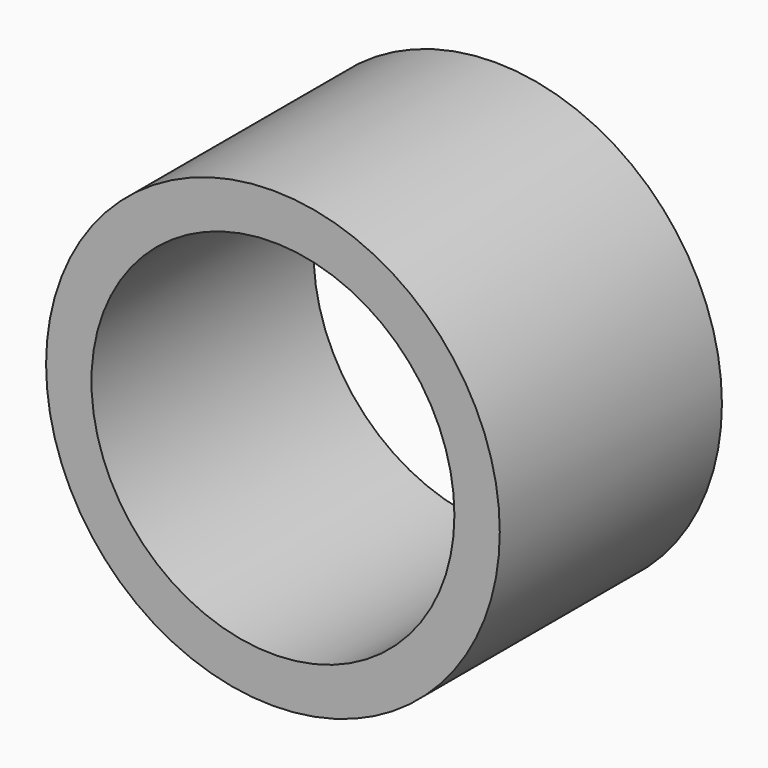
from build123d import *

# Parameters (mm, degrees)
F0_R     = 63.5
F0_R_2   = 50.8
F1_DEPTH = 77.724


# Not quite as in the source:
# - a feature names something its author has since deleted; it is built from what else it names


with BuildPart() as f1:
    # F0 (on Front) → F1 (new body)
    with BuildSketch(Plane.XZ):
        Circle(F0_R)
        Circle(F0_R_2, mode=Mode.SUBTRACT)
    extrude(amount=F1_DEPTH)


solid = f1.part
